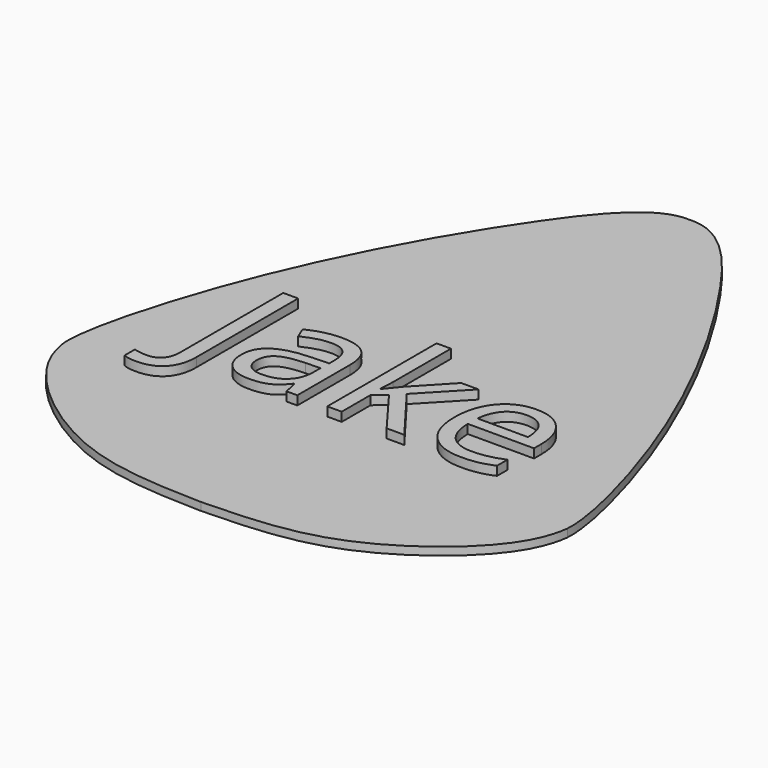
from build123d import *

# Parameters (mm, degrees)
F1_DEPTH     = 0.44
F4_TEXT_SIZE = 10.0015627442
F5_DEPTH     = 0.5


# Not quite as in the source:
# - Text() gives the source's letters only with a copy of the font that has no kerning and outlines rounded to 1/6400 em; it was checked with that copy


with BuildPart() as f1:
    # F0 (on Top) → F1 (new body)
    with BuildSketch(Plane.XY):
        with BuildLine():
            Line((0, 26), (0, 0))
            Line((0, 0), (0, -8))
            add(Edge.make_bspline(
                [(0, -8), (2.2808804072, -7.9378300476), (6.8927909358, -7.8139808089), (12.7806773832, -3.4945379032), (13.8783436269, -1.0259986157), (14, 0)],
                knots=[0, 0, 0, 0, 0.368956779, 0.7390773442, 1, 1, 1, 1], degree=3))
            add(Edge.make_bspline(
                [(14, 0), (14.1249978915, 1.4920468675), (11.8342673046, 10.3275879573), (5.7318946481, 21.4766891051), (1.7463180469, 26.108231492), (0, 26)],
                knots=[0, 0, 0, 0, 0.3295937127, 0.730781888, 1, 1, 1, 1], degree=3))
        make_face()
    extrude(amount=F1_DEPTH)

    # F2: F1 across plane


with BuildPart() as f1_1:
    add(f1.part)
    add(f1.part.mirror(Plane.YZ))

    # F4 (on face) → F5 (join)
    with BuildSketch(Plane.XY.offset(0.44)):
        with Locations((-9.8184206561, 1.7031300509)):
            Text('Jake', F4_TEXT_SIZE, font='Open Sans', text_align=(TextAlign.LEFT, TextAlign.BOTTOM))
    extrude(amount=F5_DEPTH)


solid = f1_1.part
